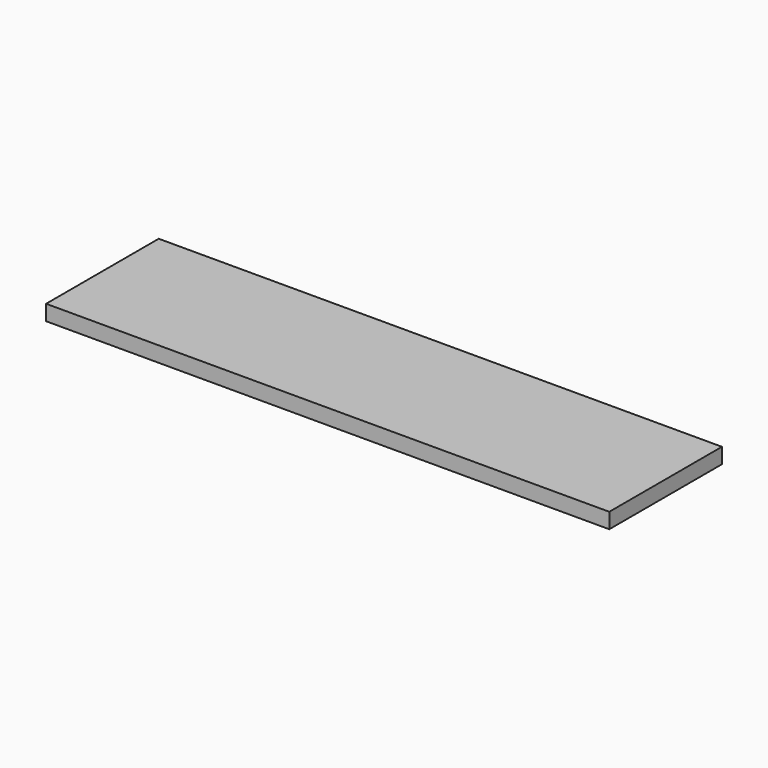
from build123d import *

# Parameters (mm, degrees)
F0_W     = 304.8
F0_H     = 8.328391239
F2_DEPTH = 76.2


# Not quite as in the source:
# - the program builds the solid bodies; features that only make, move or delete a surface that nothing else refers to are left out


with BuildPart() as f2:
    # F0 (on Front) → F2 (new body)
    with BuildSketch(Plane.XZ):
        with Locations((-198.5495146155, 32.0458719507)):
            Rectangle(F0_W, F0_H)
    extrude(amount=F2_DEPTH)


solid = f2.part
